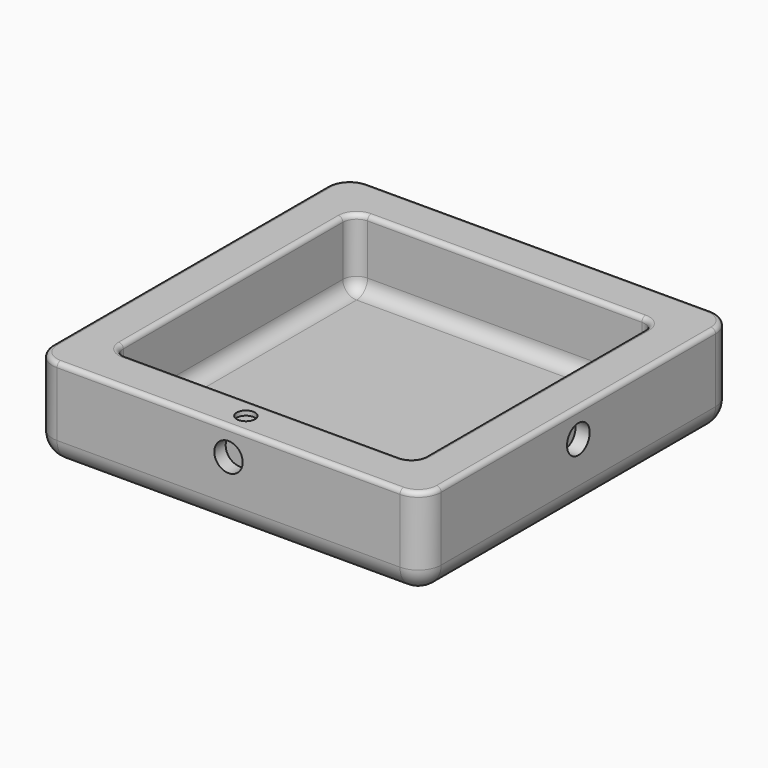
from build123d import *

# Parameters (mm, degrees)
F0_W      = 85
F0_H      = 85
F0_R      = 2
F1_DEPTH  = 20
F2_DEPTH  = 15
F3_R      = 5
F4_R      = 3
F5_R      = 1
F6_R      = 3.1
F7_DEPTH  = 3.1
F8_R      = 3.1
F9_DEPTH  = 3.1
F10_R     = 3.1
F11_DEPTH = 3.1
F12_R     = 3.1
F13_DEPTH = 3.1
F14_DEPTH = 1
F15_ANGLE = 180


# Not quite as in the source:
# - a feature names something its author has since deleted; it is built from what else it names


with BuildPart() as f1:
    # F0 (on Top) → F1 (new body)
    with BuildSketch(Plane.XY):
        Rectangle(F0_W, F0_H)
        with Locations((0, -37.75)):
            Circle(F0_R, mode=Mode.SUBTRACT)
        with BuildLine():
            ThreePointArc((-33, 30), (-32.1213203436, 32.1213203436), (-30, 33))
            Line((-30, 33), (30, 33))
            ThreePointArc((30, 33), (32.1213203436, 32.1213203436), (33, 30))
            Line((33, 30), (33, -30))
            ThreePointArc((33, -30), (32.1213203436, -32.1213203436), (30, -33))
            Line((30, -33), (-30, -33))
            ThreePointArc((-30, -33), (-32.1213203436, -32.1213203436), (-33, -30))
            Line((-33, -30), (-33, 30))
        make_face(mode=Mode.SUBTRACT)
        with BuildLine():
            Line((30, 33), (-30, 33))
            ThreePointArc((-30, 33), (-32.1213203436, 32.1213203436), (-33, 30))
            Line((-33, 30), (-33, -30))
            ThreePointArc((-33, -30), (-32.1213203436, -32.1213203436), (-30, -33))
            Line((-30, -33), (30, -33))
            ThreePointArc((30, -33), (32.1213203436, -32.1213203436), (33, -30))
            Line((33, -30), (33, 30))
            ThreePointArc((33, 30), (32.1213203436, 32.1213203436), (30, 33))
        make_face()
        with Locations((0, -37.75)):
            Circle(F0_R)
    extrude(amount=F1_DEPTH)

    # F0 (on Top) → F2 (cut)
    with BuildSketch(Plane.XY):
        with BuildLine():
            Line((30, 33), (-30, 33))
            ThreePointArc((-30, 33), (-32.1213203436, 32.1213203436), (-33, 30))
            Line((-33, 30), (-33, -30))
            ThreePointArc((-33, -30), (-32.1213203436, -32.1213203436), (-30, -33))
            Line((-30, -33), (30, -33))
            ThreePointArc((30, -33), (32.1213203436, -32.1213203436), (33, -30))
            Line((33, -30), (33, 30))
            ThreePointArc((33, 30), (32.1213203436, 32.1213203436), (30, 33))
        make_face()
    extrude(amount=F2_DEPTH, mode=Mode.SUBTRACT)

    # F3
    f3_edges = [f1.edges().sort_by_distance(p)[0] for p in [
        (0, 42.5, 20),
        (-42.5, 0, 20),
        (0, -42.5, 20),
        (42.5, 0, 20),
        (42.5, 42.5, 10),
        (-42.5, 42.5, 10),
        (-42.5, -42.5, 10),
        (42.5, -42.5, 10),
    ]]
    fillet(f3_edges, radius=F3_R)

    # F4
    f4_edges = [f1.edges().sort_by_distance(p)[0] for p in [
        (0, 33, 15),
        (-32.12132, 32.12132, 15),
        (-33, 0, 15),
        (-32.12132, -32.12132, 15),
        (0, -33, 15),
        (32.12132, -32.12132, 15),
        (33, 0, 15),
        (32.12132, 32.12132, 15),
    ]]
    fillet(f4_edges, radius=F4_R)

    # F5
    f5_edges = [f1.edges().sort_by_distance(p)[0] for p in [
        (0, 42.5, 0),
        (41.035534, 41.035534, 0),
        (-41.035534, 41.035534, 0),
        (42.5, 0, 0),
        (-42.5, 0, 0),
        (41.035534, -41.035534, 0),
        (-41.035534, -41.035534, 0),
        (0, -42.5, 0),
        (0, 33, 0),
        (-32.12132, 32.12132, 0),
        (-33, 0, 0),
        (-32.12132, -32.12132, 0),
        (0, -33, 0),
        (32.12132, -32.12132, 0),
        (33, 0, 0),
        (32.12132, 32.12132, 0),
    ]]
    fillet(f5_edges, radius=F5_R)

    # F6 (on face) → F7 (cut)
    with BuildSketch(Plane.XZ.offset(42.5)):
        with Locations((0, 6)):
            Circle(F6_R)
    extrude(amount=-F7_DEPTH, mode=Mode.SUBTRACT)

    # F8 (on face) → F9 (cut)
    with BuildSketch(Plane(origin=(0, 42.5, 0), x_dir=(-1, 0, 0), z_dir=(0, 1, 0))):
        with Locations((0, 6)):
            Circle(F8_R)
    extrude(amount=-F9_DEPTH, mode=Mode.SUBTRACT)

    # F10 (on face) → F11 (cut)
    with BuildSketch(Plane(origin=(-42.5, 0, 0), x_dir=(0, -1, 0), z_dir=(-1, 0, 0))):
        with Locations((0, 6)):
            Circle(F10_R)
    extrude(amount=-F11_DEPTH, mode=Mode.SUBTRACT)

    # F12 (on face) → F13 (cut)
    with BuildSketch(Plane.YZ.offset(42.5)):
        with Locations((0, 6)):
            Circle(F12_R)
    extrude(amount=-F13_DEPTH, mode=Mode.SUBTRACT)

    # F0 (on Top) → F14 (cut)
    with BuildSketch(Plane.XY):
        with Locations((0, -37.75)):
            Circle(F0_R)
    extrude(amount=F14_DEPTH, mode=Mode.SUBTRACT)


with BuildPart() as f1_1:
    # F15: moved
    add(f1.part.rotate(Axis((0, 0, 0), (0, 1, 0)), F15_ANGLE))


solid = f1_1.part
